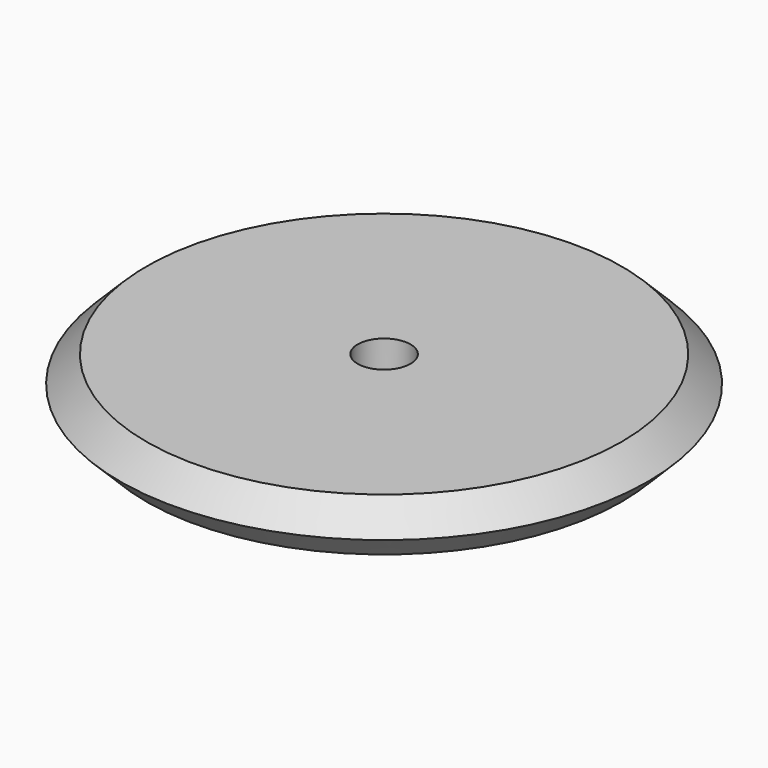
from build123d import *

# Parameters (mm, degrees)
F0_R     = 50
F0_R_2   = 40.0681224509
F0_R_3   = 5
F1_DEPTH = 5
F2_SIZE2 = 4.99999
F2_SIZE  = 4.99999


# Not quite as in the source:
# - a fillet or chamfer is up to 0.001 mm smaller than in the source, because OpenCascade refuses the exact size


with BuildPart() as f1:
    # F0 (on Top) → F1 (new body, symmetric)
    with BuildSketch(Plane.XY):
        Circle(F0_R)
        Circle(F0_R_2, mode=Mode.SUBTRACT)
        Circle(F0_R_2)
        Circle(F0_R_3, mode=Mode.SUBTRACT)
    extrude(amount=F1_DEPTH, both=True)

    # F2 (size 5 and 5 in the source; OpenCascade refuses exactly that, so slightly less here)
    f2_edges = [f1.edges().sort_by_distance(p)[0] for p in [
        (-50, 0, 5),
        (-50, 0, -5),
    ]]
    chamfer(f2_edges, length=F2_SIZE, length2=F2_SIZE2)


solid = f1.part
